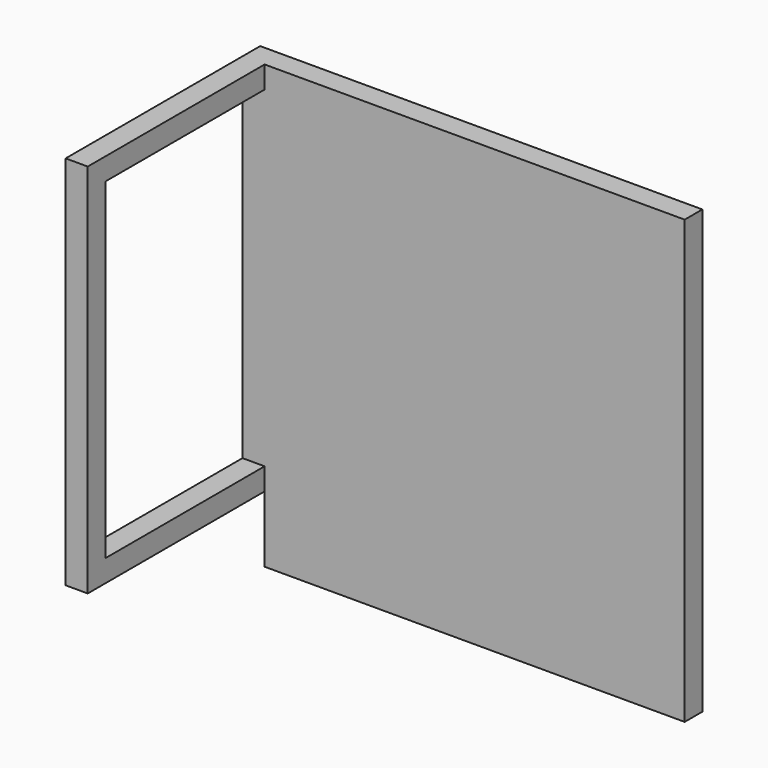
from build123d import *

# Parameters (mm, degrees)
F0_W     = 40
F0_H     = 40
F1_DEPTH = 2
F2_W     = 2
F2_H     = 34
F3_DEPTH = 20
F4_W     = 18
F4_H     = 30
F5_DEPTH = 40.001
F6_W     = 2
F6_H     = 6
F7_DEPTH = 2


# Not quite as in the source:
# - the program builds the solid bodies; features that only make, move or delete a surface that nothing else refers to are left out


with BuildPart() as f1:
    # F0 (on Front) → F1 (new body)
    with BuildSketch(Plane.XZ):
        with Locations((-31.0945767164, 25.4016729393)):
            Rectangle(F0_W, F0_H)
    extrude(amount=F1_DEPTH)

    # F2 (on face) → F3 (join)
    with BuildSketch(Plane.XZ.offset(2)):
        with Locations((-50.0945767164, 28.4016729393)):
            Rectangle(F2_W, F2_H)
    extrude(amount=F3_DEPTH)

    # F4 (on face) → F5 (cut, through all)
    with BuildSketch(Plane(origin=(-51.0945767164, 0, 0), x_dir=(0, -1, 0), z_dir=(-1, 0, 0))):
        with Locations((11, 28.4016729393)):
            Rectangle(F4_W, F4_H)
    extrude(amount=-F5_DEPTH, mode=Mode.SUBTRACT)

    # F6 (on face) → F7 (cut)
    with BuildSketch(Plane(origin=(-51.0945767164, 0, 0), x_dir=(0, -1, 0), z_dir=(-1, 0, 0))):
        with Locations((1, 8.4016729393)):
            Rectangle(F6_W, F6_H)
    extrude(amount=-F7_DEPTH, mode=Mode.SUBTRACT)


solid = f1.part
